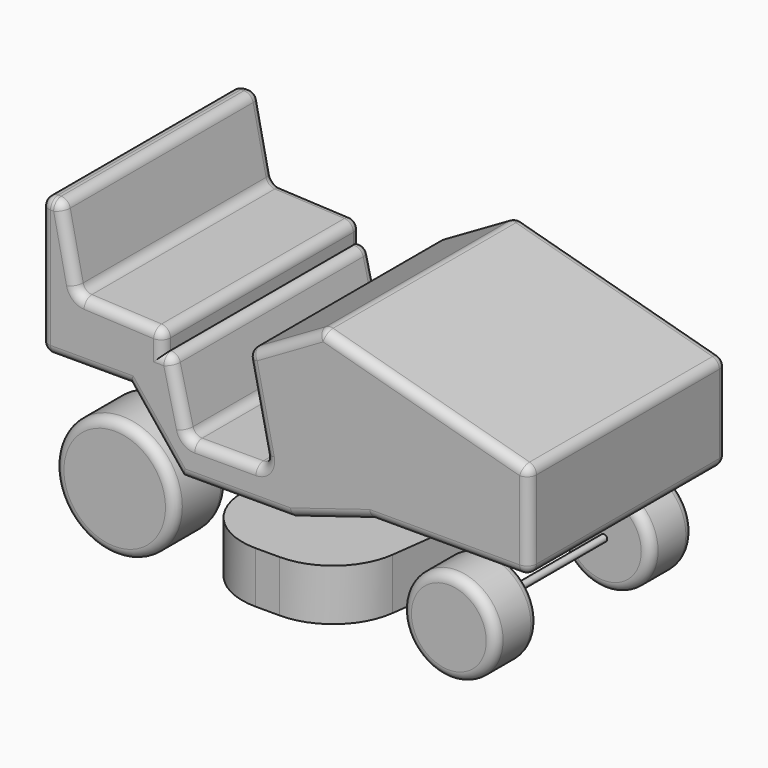
from build123d import *

# Parameters (mm, degrees)
F1_DEPTH  = 469.9
F2_R      = 38.1
F3_DEPTH  = 469.9
F2_R_2    = 12.7
F4_R      = 228.6
F5_DEPTH  = 254
F6_R      = 177.8
F7_DEPTH  = 203.2
F9_R      = 35.56
F9_2_R    = 35.56
F14_DEPTH = 195.58
F15_R     = 254


# Not quite as in the source:
# - a feature names something its author has since deleted; it is built from what else it names


with BuildPart() as f1:
    # F0 (on Front) → F1 (new body, symmetric)
    with BuildSketch(Plane.XZ):
        Polygon((247.1587508917, 439.1429820538), (847.4536012151, 439.1429820538), (847.4536012151, 800.1), (60.0536012151, 1016), (-225.9079871145, 850.9), (-146.3021296523, 482.6), (-451.1021296523, 482.6), (-512.876868248, 736.6), (-543.7560677528, 736.6), (-543.7560677528, 812.8), (-869.8304663276, 828.0904187125), (-930.5463987849, 1117.6), (-1006.7463987849, 1117.6), (-1006.7463987849, 593.5391248643), (-674.0716099739, 593.5391248643), (-475.9298563004, 346.5052941322), (-53.913731128, 346.5052941322), align=None)
    extrude(amount=F1_DEPTH, both=True)

    # F9
    f9_edges = [f1.edges().sort_by_distance(p)[0] for p in [
        (-900.188433, -469.9, 972.845209),
        (-968.646399, -469.9, 1117.6),
        (-1006.746399, -469.9, 855.569562),
        (-840.409004, -469.9, 593.539125),
        (-575.000733, -469.9, 470.022209),
        (-264.921794, -469.9, 346.505294),
        (96.62251, -469.9, 392.824138),
        (547.306176, -469.9, 439.142982),
        (847.453601, -469.9, 619.621491),
        (453.753601, -469.9, 908.05),
        (-82.927193, -469.9, 933.45),
        (-186.105058, -469.9, 666.75),
        (-298.70213, -469.9, 482.6),
        (-481.989499, -469.9, 609.6),
        (-528.316468, -469.9, 736.6),
        (-543.756068, -469.9, 774.7),
        (-706.793267, -469.9, 820.445209),
        (-900.188433, 469.9, 972.845209),
        (-968.646399, 469.9, 1117.6),
        (-1006.746399, 469.9, 855.569562),
        (-840.409004, 469.9, 593.539125),
        (-575.000733, 469.9, 470.022209),
        (-264.921794, 469.9, 346.505294),
        (96.62251, 469.9, 392.824138),
        (547.306176, 469.9, 439.142982),
        (847.453601, 469.9, 619.621491),
        (453.753601, 469.9, 908.05),
        (-82.927193, 469.9, 933.45),
        (-186.105058, 469.9, 666.75),
        (-298.70213, 469.9, 482.6),
        (-481.989499, 469.9, 609.6),
        (-528.316468, 469.9, 736.6),
        (-543.756068, 469.9, 774.7),
        (-706.793267, 469.9, 820.445209),
        (847.453601, 0, 800.1),
        (60.053601, 0, 1016),
        (847.453601, 0, 439.142982),
        (-225.907987, 0, 850.9),
        (-146.30213, 0, 482.6),
        (-451.10213, 0, 482.6),
        (-869.830466, 0, 828.090419),
        (-543.756068, 0, 812.8),
        (-930.546399, 0, 1117.6),
        (-1006.746399, 0, 1117.6),
        (-1006.746399, 0, 593.539125),
        (-512.876868, 0, 736.6),
    ]]
    fillet(f9_edges, radius=F9_R)


with BuildPart() as f3:
    # F2 (on Front) → F3 (new body, symmetric)
    with BuildSketch(Plane.XZ):
        with Locations((-727.3463987849, 228.6)):
            Circle(F2_R)
    extrude(amount=F3_DEPTH, both=True)

    # F4 (on face) → F5 (join)
    with BuildSketch(Plane.XZ.offset(469.9)):
        with Locations((-727.3463987849, 228.6)):
            Circle(F4_R)
    extrude(amount=-F5_DEPTH)



with BuildPart() as f3b:
    # F2 (on Front) → F3, piece 2 (new body, symmetric)
    with BuildSketch(Plane.XZ):
        with Locations((542.6536012151, 177.8)):
            Circle(F2_R_2)
    extrude(amount=F3_DEPTH, both=True)

    # F6 (on face) → F7 (join)
    with BuildSketch(Plane.XZ.offset(469.9)):
        with Locations((542.6536012151, 177.8)):
            Circle(F6_R)
    extrude(amount=-F7_DEPTH)


with BuildPart() as f3_1:
    add(f3.part)

    add(f3b.part)  # F8 merges F3b
    # F8: F3, F3b across plane
    add(f3.part.mirror(Plane.XZ))
    add(f3b.part.mirror(Plane.XZ))

    # F9#2
    f9_2_edges = [f3_1.edges().sort_by_distance(p)[0] for p in [
        (-498.746399, -342.9, 228.6),
        (-955.946399, -469.9, 228.6),
        (-955.946399, -215.9, 228.6),
        (-498.746399, 342.9, 228.6),
        (-955.946399, 469.9, 228.6),
        (-955.946399, 215.9, 228.6),
        (720.453601, -368.3, 177.8),
        (364.853601, -469.9, 177.8),
        (364.853601, -266.7, 177.8),
        (720.453601, 368.3, 177.8),
        (364.853601, 469.9, 177.8),
        (364.853601, 266.7, 177.8),
    ]]
    fillet(f9_2_edges, radius=F9_2_R)


with BuildPart() as f14:
    # F13 (on offset) → F14 (new body)
    with BuildSketch(Plane.XY.offset(50.8)):
        Polygon((312.7593517316, 533.4), (-308.6305973146, 533.4), (-423.5990158775, -533.4), (173.7277868513, -533.4), align=None)
    extrude(amount=F14_DEPTH)

    # F15
    f15_edges = [f14.edges().sort_by_distance(p)[0] for p in [
        (173.727787, -533.4, 148.59),
        (-423.599016, -533.4, 148.59),
        (312.759352, 533.4, 148.59),
        (-308.630597, 533.4, 148.59),
    ]]
    fillet(f15_edges, radius=F15_R)


solid = Compound([f1.part, f3_1.part, f14.part])
